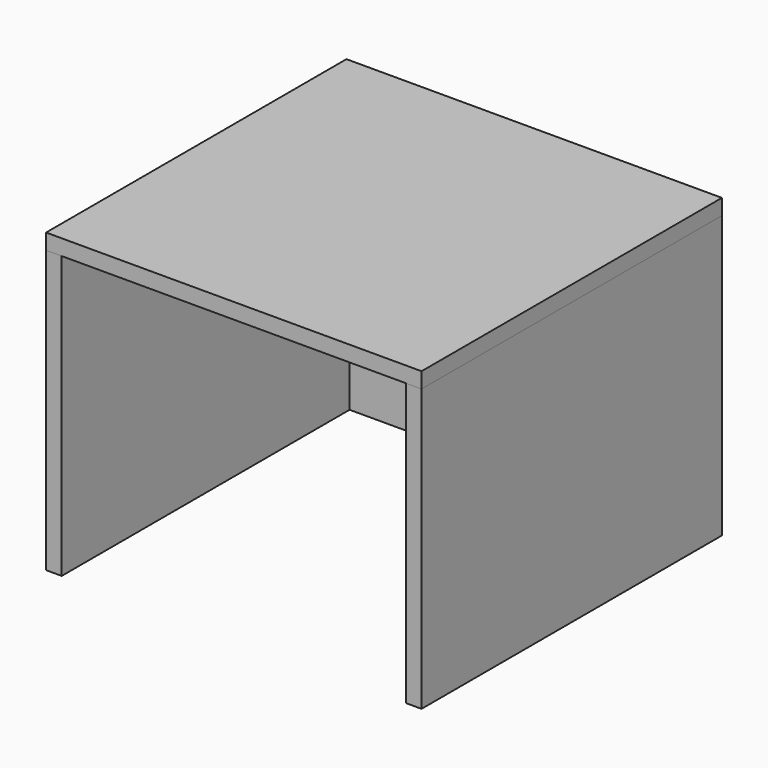
from build123d import *

# Parameters (mm, degrees)
F0_W     = 609.6
F0_H     = 609.6
F1_DEPTH = 25.4
F2_W     = 609.6
F2_H     = 457.2
F3_DEPTH = 25.4
F4_W     = 609.6
F4_H     = 457.2
F5_DEPTH = 25.4
F6_W     = 558.8
F6_H     = 457.2
F7_DEPTH = 25.4


with BuildPart() as f1:
    # F0 (on Top) → F1 (new body)
    with BuildSketch(Plane.XY):
        with Locations((304.8, -304.8)):
            Rectangle(F0_W, F0_H)
    extrude(amount=F1_DEPTH)


with BuildPart() as f3:
    # F2 (on face) → F3 (new body)
    with BuildSketch(Plane.YZ.offset(609.6)):
        with Locations((-304.8, -228.6)):
            Rectangle(F2_W, F2_H)
    extrude(amount=-F3_DEPTH)


with BuildPart() as f5:
    # F4 (on face) → F5 (new body)
    with BuildSketch(Plane(origin=(0, 0, 0), x_dir=(0, -1, 0), z_dir=(-1, 0, 0))):
        with Locations((304.8, -228.6)):
            Rectangle(F4_W, F4_H)
    extrude(amount=-F5_DEPTH)

    # F6 (on face) → F7 (join)
    with BuildSketch(Plane(origin=(0, 0, 0), x_dir=(-1, 0, 0), z_dir=(0, 1, 0))):
        with Locations((-304.7380357742, -228.6)):
            Rectangle(F6_W, F6_H)
    extrude(amount=-F7_DEPTH)


solid = Compound([f1.part, f3.part, f5.part])
